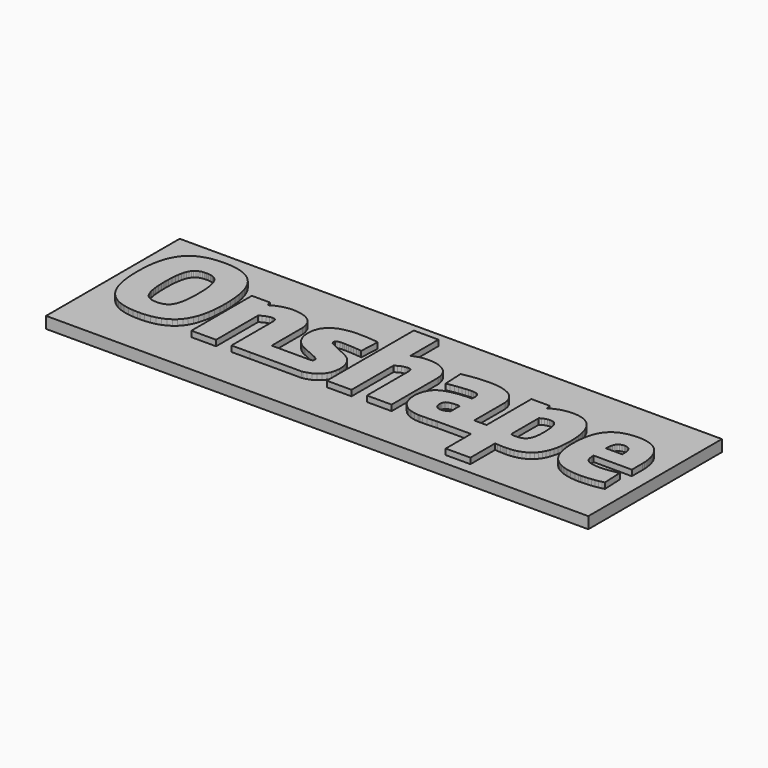
from build123d import *

# Parameters (mm, degrees)
F4_DEPTH = 21.0730088496
F3_W     = 659.7553988
F3_H     = 203.2
F5_DEPTH = 14.0486725664
F6_SCALE = 0.226


# Not quite as in the source:
# - a length typed as a fraction of an inch, garbled in the dataset ("3 / 203.2 mm" for 3/8 in), is restored


with BuildPart() as f4:
    # F3 (on Top) → F4 (new body)
    with BuildSketch(Plane.XY):
        Polygon((-255.4416786, 81.57591), (-257.1904686, 81.57591), (-258.9486566, 81.57591), (-264.2209346, 81.33461), (-270.6951406, 80.60309), (-276.6260406, 79.37881), (-282.0281126, 77.65669), (-286.9158346, 75.43165), (-291.3049546, 72.69861), (-295.2061406, 69.44995), (-298.637579, 65.68567), (-301.6113856, 61.39561), (-304.1428258, 56.57977), (-306.2443456, 51.22799), (-307.9324296, 45.34281), (-309.2209208, 38.91153), (-310.1235352, 31.93415), (-310.654065, 24.40305), (-310.8276994, 18.33753), (-310.8276994, 16.31315), (-310.8276994, 14.29131), (-310.654065, 8.22833), (-310.1235352, 0.70231), (-309.2209208, -6.26491), (-307.9324296, -12.68603), (-306.2443456, -18.55851), (-304.1428258, -23.88997), (-301.6113856, -28.69057), (-298.637579, -32.96285), (-295.2061406, -36.70935), (-291.3049546, -39.94023), (-286.9158346, -42.65803), (-282.0281126, -44.86783), (-276.6260406, -46.57979), (-270.6951406, -47.79645), (-264.2209346, -48.52035), (-258.9486566, -48.75911), (-257.1904686, -48.75911), (-255.4416786, -48.75911), (-250.1953086, -48.52035), (-243.7569166, -47.79645), (-237.8608146, -46.57979), (-232.4917626, -44.86783), (-227.6355366, -42.65803), (-223.2781666, -39.94023), (-219.4059366, -36.70935), (-216.0023366, -32.96285), (-213.0531426, -28.69057), (-210.5451466, -23.88997), (-208.4631086, -18.55851), (-206.7912806, -12.68603), (-205.5167086, -6.26491), (-204.6251686, 0.70231), (-204.0998966, 8.22833), (-203.9276846, 14.29131), (-203.9276846, 16.31315), (-203.9276846, 18.33753), (-204.0998966, 24.40305), (-204.6251686, 31.93415), (-205.5167086, 38.91153), (-206.7912806, 45.34281), (-208.4631086, 51.22799), (-210.5451466, 56.57977), (-213.0531426, 61.39561), (-216.0023366, 65.68567), (-219.4059366, 69.44995), (-223.2781666, 72.69861), (-227.6355366, 75.43165), (-232.4917626, 77.65669), (-237.8608146, 79.37881), (-243.7569166, 80.60309), (-250.1953086, 81.33461), align=None)
        Polygon((-256.5633426, -21.56841), (-257.1904686, -21.56841), (-257.8269926, -21.56841), (-259.7342786, -21.48205), (-262.0906366, -21.20773), (-264.2651306, -20.72513), (-266.2592846, -20.00123), (-268.0769086, -19.01317), (-269.7207966, -17.74063), (-271.1924726, -16.15313), (-272.4975246, -14.23035), (-273.6387466, -11.94435), (-274.6156306, -9.26973), (-275.4352886, -6.18363), (-276.0997526, -2.65811), (-276.6095306, 1.32715), (-276.9707186, 5.80517), (-277.1856026, 10.78865), (-277.2557066, 14.93393), (-277.2557066, 16.31315), (-277.2557066, 17.69745), (-277.1856026, 21.84019), (-276.9707186, 26.83383), (-276.6095306, 31.31947), (-276.0997526, 35.31743), (-275.4352886, 38.85565), (-274.6156306, 41.95953), (-273.6387466, 44.64939), (-272.4975246, 46.95571), (-271.1924726, 48.89627), (-269.7207966, 50.49647), (-268.0769086, 51.78933), (-266.2592846, 52.79009), (-264.2651306, 53.52415), (-262.0906366, 54.01945), (-259.7342786, 54.29631), (-257.8269926, 54.38521), (-257.1904686, 54.38521), (-256.5633426, 54.38521), (-254.6779006, 54.30139), (-252.3436406, 54.02453), (-250.1856566, 53.53939), (-248.1998846, 52.81549), (-246.3865786, 51.82489), (-244.7424366, 50.54727), (-243.2651726, 48.95469), (-241.9519926, 47.02683), (-240.8023886, 44.73067), (-239.8133126, 42.04081), (-238.9822246, 38.93947), (-238.3070926, 35.39617), (-237.7861386, 31.38805), (-237.4168226, 26.88971), (-237.1963506, 21.87321), (-237.1234526, 17.70253), (-237.1234526, 16.31315), (-237.1234526, 14.92631), (-237.1963506, 10.75817), (-237.4168226, 5.74675), (-237.7861386, 1.25603), (-238.3070926, -2.73685), (-238.9822246, -6.26491), (-239.8133126, -9.35101), (-240.8023886, -12.02055), (-241.9519926, -14.30147), (-243.2651726, -16.21663), (-244.7424366, -17.78889), (-246.3865786, -19.05381), (-248.1998846, -20.02663), (-250.1856566, -20.73783), (-252.3436406, -21.21789), (-254.6779006, -21.48205), align=None, mode=Mode.SUBTRACT)
    extrude(amount=F4_DEPTH)



with BuildPart() as f4b:
    # F3 (on Top) → F4, piece 2 (new body)
    with BuildSketch(Plane.XY):
        Polygon((-50.1012206, 5.24383), (-50.9191006, 5.62483), (-70.0513966, 14.62659), (-70.5279006, 14.84503), (-71.9403946, 15.54353), (-73.3544126, 16.47825), (-74.2421426, 17.66189), (-74.5479586, 18.90141), (-74.5479586, 19.31543), (-74.5479586, 19.75993), (-74.1148886, 21.09089), (-72.6284806, 22.24659), (-69.8040006, 22.87397), (-66.4715206, 23.06447), (-65.3615406, 23.06447), (-65.0237206, 23.06447), (-64.0026406, 23.04669), (-61.8690406, 22.98827), (-59.1360006, 22.87905), (-55.9838606, 22.71649), (-52.5853406, 22.49043), (-49.1157006, 22.19833), (-45.7527406, 21.82749), (-43.4362606, 21.50999), (-42.6691806, 21.38045), (-41.5439606, 45.19549), (-42.3059606, 45.32503), (-44.5995806, 45.64761), (-47.9142806, 46.01337), (-51.3610606, 46.30547), (-54.8129206, 46.53153), (-58.1403206, 46.69409), (-61.2188006, 46.80331), (-63.9188206, 46.86427), (-65.5622006, 46.88205), (-66.1108406, 46.88205), (-68.1606206, 46.88205), (-74.3025946, 46.52137), (-81.7783226, 45.38853), (-88.4247406, 43.42003), (-94.1227226, 40.55745), (-98.7587306, 36.71697), (-102.2133846, 31.85033), (-104.3726386, 25.88387), (-105.1168586, 20.53717), (-105.1168586, 18.75155), (-105.1168586, 17.49933), (-104.7681166, 13.73759), (-103.7663406, 9.23671), (-102.1803646, 5.23367), (-100.0772446, 1.71069), (-97.5253066, -1.34747), (-94.5941466, -3.95351), (-91.3503126, -6.12267), (-88.7567186, -7.49173), (-87.8623846, -7.87781), (-70.6122286, -15.56639), (-70.0513966, -15.81531), (-68.4273206, -16.69669), (-66.9084006, -17.86255), (-66.0244806, -19.10207), (-65.7374606, -20.10791), (-65.7374606, -20.44319), (-65.7374606, -20.68957), (-65.8314406, -21.42617), (-66.1337006, -22.15769), (-66.6823406, -22.66823), (-67.5129206, -23.00097), (-68.6610006, -23.19401), (-70.1588386, -23.28545), (-72.0452966, -23.31085), (-73.7773226, -23.31085), (-74.3533946, -23.31085), (-75.5360186, -23.31085), (-79.0790646, -23.31085), (-85.2952066, -23.31085), (-92.4722306, -23.31339), (-98.1758006, -23.31847), (-100.0759746, -23.32101), (-100.0759746, -23.31085), (-115.8120366, -23.31085), (-115.8120366, 22.12721), (-115.8120366, 23.76805), (-116.5024086, 28.68549), (-118.4493186, 34.06521), (-121.4686166, 38.36797), (-125.3769146, 41.68267), (-129.9875226, 44.09567), (-135.1165446, 45.70603), (-140.5808466, 46.60265), (-144.7906426, 46.88205), (-146.1934846, 46.88205), (-147.9712306, 46.88205), (-153.3026906, 46.28769), (-159.8840846, 44.65447), (-165.7631686, 42.21353), (-169.5787566, 40.04437), (-170.7598566, 39.19347), (-170.9485786, 39.19347), (-172.6338686, 45.00499), (-194.5776906, 45.00499), (-194.5776906, -46.88205), (-164.5711466, -46.88205), (-164.5711466, 16.87703), (-163.7926366, 17.44599), (-161.3021666, 18.93443), (-157.8200806, 20.53717), (-154.3392646, 21.57349), (-151.8863866, 21.93925), (-151.0674906, 21.93925), (-150.7421166, 21.93925), (-149.7654866, 21.87067), (-148.6656666, 21.64969), (-147.7588866, 21.26869), (-147.0367646, 20.72259), (-146.4899026, 19.99869), (-146.1106806, 19.09445), (-145.8902086, 17.99209), (-145.8170566, 17.01927), (-145.8170566, 16.69161), (-145.8170566, -46.88205), (-123.4378786, -46.88205), (-60.4542606, -46.92523), (-59.1131406, -46.68901), (-55.1405806, -45.67047), (-50.3272806, -43.85183), (-46.0753206, -41.43629), (-42.4558206, -38.38829), (-39.5272006, -34.66973), (-37.3529606, -30.24759), (-36.0042206, -25.07869), (-35.5394006, -20.61591), (-35.5394006, -19.13001), (-35.5394006, -17.97685), (-35.8391206, -14.51991), (-36.7027206, -10.38479), (-38.0819406, -6.69925), (-39.9234406, -3.44551), (-42.1815006, -0.60579), (-44.7977006, 1.83769), (-47.7288606, 3.91033), align=None)
    extrude(amount=F4_DEPTH)


with BuildPart() as f4c:
    # F3 (on Top) → F4, piece 3 (new body)
    with BuildSketch(Plane.XY):
        Polygon((19.9824594, 46.88459), (18.5778394, 46.88459), (17.3408594, 46.88459), (13.6248394, 46.57725), (8.7785194, 45.71365), (4.2827194, 44.35221), (1.3185394, 43.09237), (0.3863594, 42.57167), (0.1983994, 42.57167), (0.1983994, 85.33003), (-29.8091606, 85.33003), (-29.8091606, -46.88205), (0.1983994, -46.88205), (0.1983994, 16.87703), (0.9781794, 17.44599), (3.4673794, 18.93443), (6.9497194, 20.53717), (10.4295194, 21.57349), (12.8806194, 21.93925), (13.7010394, 21.93925), (14.0261594, 21.93925), (15.0015194, 21.87067), (16.1013394, 21.64969), (17.0106594, 21.26869), (17.7320194, 20.72259), (18.2781194, 19.99869), (18.6591194, 19.09445), (18.8800994, 17.99717), (18.9512194, 17.01927), (18.9512194, 16.69161), (18.9512194, -46.88205), (48.9613194, -46.88205), (48.9613194, 22.12721), (48.9613194, 23.76805), (48.2678994, 28.68549), (46.3222594, 34.06521), (43.3021994, 38.36797), (39.3931394, 41.68267), (34.7830394, 44.09567), (29.6522394, 45.70603), (24.1912394, 46.60519), align=None)
    extrude(amount=F4_DEPTH)


with BuildPart() as f4d:
    # F3 (on Top) → F4, piece 4 (new body)
    with BuildSketch(Plane.XY):
        Polygon((196.4946794, 46.88459), (195.2983394, 46.88459), (193.6498794, 46.88459), (188.6994194, 46.50105), (181.8668194, 45.22089), (175.2831394, 42.84853), (170.7466994, 40.27805), (169.4208194, 39.19347), (169.2328594, 39.19347), (167.5437594, 45.00753), (145.6006994, 45.00753), (145.6006994, -23.32101), (130.5969194, -23.32101), (130.5969194, 21.75383), (130.5969194, 23.36927), (129.8171394, 28.21559), (127.5870194, 33.59277), (124.0818194, 37.94633), (119.4640994, 41.34993), (113.9040394, 43.87977), (107.5743594, 45.59427), (100.6426994, 46.57471), (95.1181994, 46.88459), (93.2766994, 46.88459), (91.5469594, 46.88459), (86.3628194, 46.66615), (78.1763994, 45.99305), (69.4362594, 44.82465), (62.9617994, 43.63847), (60.8307394, 43.13047), (61.9559594, 18.94205), (63.1268994, 19.18843), (66.6651194, 19.84883), (71.3133194, 20.60321), (75.7862594, 21.22043), (79.9823394, 21.70811), (83.8050394, 22.06625), (87.1451394, 22.31517), (89.8959594, 22.45995), (91.4478994, 22.50059), (91.9635194, 22.50059), (92.9312594, 22.50059), (95.8243194, 22.18309), (98.6462594, 21.07565), (100.3785394, 18.94459), (100.9678194, 16.40967), (100.9678194, 15.56639), (100.9678194, 10.49909), (99.6216194, 10.49909), (95.5982594, 10.40511), (90.0102594, 10.09015), (84.3765394, 9.50595), (78.8571194, 8.60425), (73.6323394, 7.34187), (68.8672994, 5.67817), (64.7321794, 3.55727), (62.1413794, 1.68275), (61.3946194, 0.93599), (60.4116394, -0.04445), (57.9554594, -3.49123), (55.6948594, -8.46201), (54.4553394, -13.75029), (54.0794194, -17.78635), (54.0794194, -19.13001), (54.0794194, -20.80133), (54.6585394, -25.83053), (56.3222394, -31.59125), (58.9663794, -36.43503), (62.4715794, -40.37711), (66.7362394, -43.44035), (71.6435194, -45.64253), (77.0867394, -46.99635), (81.4910994, -47.49419), (82.9617594, -47.52467), (83.9980794, -47.54245), (87.1095794, -47.53229), (92.3343594, -47.42307), (98.3312994, -47.20463), (103.1750794, -46.97095), (104.7879794, -46.87951), (145.6006994, -46.88967), (145.6006994, -85.33003), (175.6082594, -85.33003), (175.6082594, -47.63389), (176.3829594, -47.75073), (178.7400794, -47.99203), (182.2655994, -48.22063), (185.7885794, -48.34763), (188.1380794, -48.38573), (188.9254794, -48.38573), (190.1573794, -48.38573), (193.8505394, -48.20031), (198.4403194, -47.63897), (202.6897394, -46.69917), (206.6089594, -45.38853), (210.1979794, -43.69689), (213.4542594, -41.62933), (216.3930394, -39.18585), (219.0016194, -36.35883), (221.2952394, -33.15335), (223.2738994, -29.56941), (224.9401394, -25.59939), (226.2939594, -21.25091), (227.3455194, -16.51381), (228.0897394, -11.39317), (228.5342394, -5.89153), (228.6866394, -1.47447), (228.6866394, -0.00381), (228.6866394, 1.17475), (228.6053594, 4.69519), (228.3513594, 9.28243), (227.8992394, 13.72743), (227.2413794, 18.00733), (226.3447594, 22.09165), (225.1915994, 25.95753), (223.7691994, 29.58211), (222.0470794, 32.93745), (220.0150794, 35.99053), (217.6477994, 38.72611), (214.9249194, 41.11117), (211.8311994, 43.12031), (208.3386994, 44.72559), (204.4321794, 45.90669), (200.0938594, 46.63567), align=None)
        Polygon((101.3361194, -8.62711), (101.3361194, -22.50567), (100.8890794, -22.91461), (99.3193594, -23.90267), (96.8606394, -24.96439), (94.3003194, -25.64257), (92.5451794, -25.88133), (91.9635194, -25.88133), (91.0465794, -25.88133), (88.2982994, -25.31745), (85.7278194, -23.63089), (84.2063594, -20.81657), (83.7085194, -17.86255), (83.7085194, -16.87957), (83.7085194, -16.62557), (83.7643994, -15.87119), (84.0158594, -14.44117), (84.5797394, -12.86891), (85.2833194, -11.74369), (85.5855794, -11.43889), (86.1011994, -10.92581), (88.1535194, -9.89203), (91.7730194, -9.04875), (96.2408794, -8.69823), (100.0635794, -8.62711), align=None, mode=Mode.SUBTRACT)
        Polygon((185.2780394, -24.04745), (184.4245994, -24.12619), (183.8835794, -24.17191), (182.2579794, -24.21255), (179.8805394, -24.12873), (177.5665994, -23.86203), (176.0806994, -23.55723), (175.6082594, -23.39975), (175.6082594, 18.56867), (176.1060994, 18.95221), (177.7342394, 19.94281), (180.3885394, 21.14677), (183.4670194, 21.99767), (186.0146394, 22.31771), (186.8604594, 22.31771), (187.4878394, 22.31771), (189.3648994, 22.10181), (191.5391394, 21.36775), (193.3780994, 19.98599), (194.8766994, 17.81683), (196.0476394, 14.73581), (196.8807594, 10.60831), (197.3811394, 5.30225), (197.5462394, 0.33909), (197.5462394, -1.31445), (197.5462394, -2.68097), (197.3887594, -6.78053), (196.8832994, -11.40079), (195.9942994, -15.22603), (194.6811194, -18.30197), (192.9107394, -20.67941), (190.6348994, -22.40661), (187.8180394, -23.53945), align=None, mode=Mode.SUBTRACT)
    extrude(amount=F4_DEPTH)


with BuildPart() as f4e:
    # F3 (on Top) → F4, piece 5 (new body)
    with BuildSketch(Plane.XY):
        Polygon((276.0119194, 46.88459), (274.8181194, 46.88459), (273.3982594, 46.88459), (269.1285194, 46.67377), (263.9316794, 46.04893), (259.2098194, 45.01515), (254.9426194, 43.58005), (251.1199194, 41.74871), (247.7188594, 39.52621), (244.7241994, 36.92271), (242.1156194, 33.94583), (239.8829594, 30.59811), (238.0033594, 26.88717), (236.4590394, 22.81809), (235.2347594, 18.40103), (234.3127394, 13.64361), (233.6751994, 8.54837), (233.3043594, 3.12293), (233.1849794, -1.19253), (233.1849794, -2.62763), (233.1849794, -3.94081), (233.3221394, -7.87273), (233.7463194, -12.84859), (234.4727594, -17.53997), (235.5166994, -21.93925), (236.9035394, -26.03881), (238.6459794, -29.83103), (240.7592594, -33.30575), (243.2662394, -36.45281), (246.1796194, -39.26459), (249.5222594, -41.72839), (253.3068594, -43.83913), (257.5537394, -45.58411), (262.2806794, -46.96079), (267.5029194, -47.95647), (273.2382394, -48.55591), (277.9423194, -48.75911), (279.5069594, -48.75911), (280.1927594, -48.75911), (282.2374594, -48.70831), (285.5343794, -48.54575), (289.2122994, -48.27651), (293.1035794, -47.89297), (297.0304194, -47.39513), (300.8200994, -46.78045), (304.2871994, -46.05147), (306.5300194, -45.44695), (307.2640794, -45.20057), (306.1363194, -21.19503), (304.9780794, -21.52269), (301.4474794, -22.32279), (295.7527994, -23.34895), (289.8117394, -24.09317), (285.7401194, -24.38273), (284.3837594, -24.38273), (282.8495994, -24.38273), (278.2445794, -24.12873), (273.4973194, -23.37435), (269.9590994, -22.12467), (267.4571994, -20.39747), (265.8188994, -18.18767), (264.8663994, -15.51813), (264.4218994, -12.39139), (264.3177594, -9.70661), (264.3177594, -8.81507), (310.8276994, -8.81507), (310.8276994, 6.56209), (310.8276994, 7.61619), (310.7133994, 10.78611), (310.3654194, 14.86281), (309.7685194, 18.77949), (308.9176194, 22.51583), (307.8000194, 26.05405), (306.4080994, 29.37637), (304.7240794, 32.46755), (302.7377994, 35.30219), (300.4441794, 37.87521), (297.8305194, 40.15867), (294.8891994, 42.13987), (291.5998994, 43.80103), (287.9600794, 45.12437), (283.9595794, 46.09211), (279.5806194, 46.68393), align=None)
        Polygon((284.0129194, 11.81481), (284.0129194, 10.12571), (264.1297994, 10.12571), (264.1628194, 10.91311), (264.3279194, 13.26515), (264.6936794, 16.16837), (265.3108994, 18.78203), (266.2608594, 21.05025), (267.6248394, 22.91461), (269.4815794, 24.31415), (271.9148994, 25.19553), (274.2339194, 25.50287), (275.0086194, 25.50287), (275.6563194, 25.50287), (277.6019594, 25.19299), (279.6568194, 24.31415), (281.2366994, 22.95271), (282.3923994, 21.19249), (283.1899594, 19.11477), (283.6852594, 16.80337), (283.9417994, 14.34211), (284.0129194, 12.44727), align=None, mode=Mode.SUBTRACT)
    extrude(amount=F4_DEPTH)


with BuildPart() as f4_1:
    add(f4.part)

    add(f4b.part)  # F5 merges F4b

    add(f4c.part)  # F5 merges F4c

    add(f4d.part)  # F5 merges F4d

    add(f4e.part)  # F5 merges F4e
    # F3 (on Top) → F5 (join)
    with BuildSketch(Plane.XY):
        with Locations((0, 2.78003)):
            Rectangle(F3_W, F3_H)
        Polygon((-70.0513966, 14.62659), (-50.9191006, 5.62483), (-50.1012206, 5.24383), (-47.7288606, 3.91033), (-44.7977006, 1.83769), (-42.1815006, -0.60579), (-39.9234406, -3.44551), (-38.0819406, -6.69925), (-36.7027206, -10.38479), (-35.8391206, -14.51991), (-35.5394006, -17.97685), (-35.5394006, -19.13001), (-35.5394006, -20.61591), (-36.0042206, -25.07869), (-37.3529606, -30.24759), (-39.5272006, -34.66973), (-42.4558206, -38.38829), (-46.0753206, -41.43629), (-50.3272806, -43.85183), (-55.1405806, -45.67047), (-59.1131406, -46.68901), (-60.4542606, -46.92523), (-123.4378786, -46.88205), (-145.8170566, -46.88205), (-145.8170566, 16.69161), (-145.8170566, 17.01927), (-145.8902086, 17.99209), (-146.1106806, 19.09445), (-146.4899026, 19.99869), (-147.0367646, 20.72259), (-147.7588866, 21.26869), (-148.6656666, 21.64969), (-149.7654866, 21.87067), (-150.7421166, 21.93925), (-151.0674906, 21.93925), (-151.8863866, 21.93925), (-154.3392646, 21.57349), (-157.8200806, 20.53717), (-161.3021666, 18.93443), (-163.7926366, 17.44599), (-164.5711466, 16.87703), (-164.5711466, -46.88205), (-194.5776906, -46.88205), (-194.5776906, 45.00499), (-172.6338686, 45.00499), (-170.9485786, 39.19347), (-170.7598566, 39.19347), (-169.5787566, 40.04437), (-165.7631686, 42.21353), (-159.8840846, 44.65447), (-153.3026906, 46.28769), (-147.9712306, 46.88205), (-146.1934846, 46.88205), (-144.7906426, 46.88205), (-140.5808466, 46.60265), (-135.1165446, 45.70603), (-129.9875226, 44.09567), (-125.3769146, 41.68267), (-121.4686166, 38.36797), (-118.4493186, 34.06521), (-116.5024086, 28.68549), (-115.8120366, 23.76805), (-115.8120366, 22.12721), (-115.8120366, -23.31085), (-100.0759746, -23.31085), (-100.0759746, -23.32101), (-98.1758006, -23.31847), (-92.4722306, -23.31339), (-85.2952066, -23.31085), (-79.0790646, -23.31085), (-75.5360186, -23.31085), (-74.3533946, -23.31085), (-73.7773226, -23.31085), (-72.0452966, -23.31085), (-70.1588386, -23.28545), (-68.6610006, -23.19401), (-67.5129206, -23.00097), (-66.6823406, -22.66823), (-66.1337006, -22.15769), (-65.8314406, -21.42617), (-65.7374606, -20.68957), (-65.7374606, -20.44319), (-65.7374606, -20.10791), (-66.0244806, -19.10207), (-66.9084006, -17.86255), (-68.4273206, -16.69669), (-70.0513966, -15.81531), (-70.6122286, -15.56639), (-87.8623846, -7.87781), (-88.7567186, -7.49173), (-91.3503126, -6.12267), (-94.5941466, -3.95351), (-97.5253066, -1.34747), (-100.0772446, 1.71069), (-102.1803646, 5.23367), (-103.7663406, 9.23671), (-104.7681166, 13.73759), (-105.1168586, 17.49933), (-105.1168586, 18.75155), (-105.1168586, 20.53717), (-104.3726386, 25.88387), (-102.2133846, 31.85033), (-98.7587306, 36.71697), (-94.1227226, 40.55745), (-88.4247406, 43.42003), (-81.7783226, 45.38853), (-74.3025946, 46.52137), (-68.1606206, 46.88205), (-66.1108406, 46.88205), (-65.5622006, 46.88205), (-63.9188206, 46.86427), (-61.2188006, 46.80331), (-58.1403206, 46.69409), (-54.8129206, 46.53153), (-51.3610606, 46.30547), (-47.9142806, 46.01337), (-44.5995806, 45.64761), (-42.3059606, 45.32503), (-41.5439606, 45.19549), (-42.6691806, 21.38045), (-43.4362606, 21.50999), (-45.7527406, 21.82749), (-49.1157006, 22.19833), (-52.5853406, 22.49043), (-55.9838606, 22.71649), (-59.1360006, 22.87905), (-61.8690406, 22.98827), (-64.0026406, 23.04669), (-65.0237206, 23.06447), (-65.3615406, 23.06447), (-66.4715206, 23.06447), (-69.8040006, 22.87397), (-72.6284806, 22.24659), (-74.1148886, 21.09089), (-74.5479586, 19.75993), (-74.5479586, 19.31543), (-74.5479586, 18.90141), (-74.2421426, 17.66189), (-73.3544126, 16.47825), (-71.9403946, 15.54353), (-70.5279006, 14.84503), align=None, mode=Mode.SUBTRACT)
        Polygon((193.6498794, 46.88459), (195.2983394, 46.88459), (196.4946794, 46.88459), (200.0938594, 46.63567), (204.4321794, 45.90669), (208.3386994, 44.72559), (211.8311994, 43.12031), (214.9249194, 41.11117), (217.6477994, 38.72611), (220.0150794, 35.99053), (222.0470794, 32.93745), (223.7691994, 29.58211), (225.1915994, 25.95753), (226.3447594, 22.09165), (227.2413794, 18.00733), (227.8992394, 13.72743), (228.3513594, 9.28243), (228.6053594, 4.69519), (228.6866394, 1.17475), (228.6866394, -0.00381), (228.6866394, -1.47447), (228.5342394, -5.89153), (228.0897394, -11.39317), (227.3455194, -16.51381), (226.2939594, -21.25091), (224.9401394, -25.59939), (223.2738994, -29.56941), (221.2952394, -33.15335), (219.0016194, -36.35883), (216.3930394, -39.18585), (213.4542594, -41.62933), (210.1979794, -43.69689), (206.6089594, -45.38853), (202.6897394, -46.69917), (198.4403194, -47.63897), (193.8505394, -48.20031), (190.1573794, -48.38573), (188.9254794, -48.38573), (188.1380794, -48.38573), (185.7885794, -48.34763), (182.2655994, -48.22063), (178.7400794, -47.99203), (176.3829594, -47.75073), (175.6082594, -47.63389), (175.6082594, -85.33003), (145.6006994, -85.33003), (145.6006994, -46.88967), (104.7879794, -46.87951), (103.1750794, -46.97095), (98.3312994, -47.20463), (92.3343594, -47.42307), (87.1095794, -47.53229), (83.9980794, -47.54245), (82.9617594, -47.52467), (81.4910994, -47.49419), (77.0867394, -46.99635), (71.6435194, -45.64253), (66.7362394, -43.44035), (62.4715794, -40.37711), (58.9663794, -36.43503), (56.3222394, -31.59125), (54.6585394, -25.83053), (54.0794194, -20.80133), (54.0794194, -19.13001), (54.0794194, -17.78635), (54.4553394, -13.75029), (55.6948594, -8.46201), (57.9554594, -3.49123), (60.4116394, -0.04445), (61.3946194, 0.93599), (62.1413794, 1.68275), (64.7321794, 3.55727), (68.8672994, 5.67817), (73.6323394, 7.34187), (78.8571194, 8.60425), (84.3765394, 9.50595), (90.0102594, 10.09015), (95.5982594, 10.40511), (99.6216194, 10.49909), (100.9678194, 10.49909), (100.9678194, 15.56639), (100.9678194, 16.40967), (100.3785394, 18.94459), (98.6462594, 21.07565), (95.8243194, 22.18309), (92.9312594, 22.50059), (91.9635194, 22.50059), (91.4478994, 22.50059), (89.8959594, 22.45995), (87.1451394, 22.31517), (83.8050394, 22.06625), (79.9823394, 21.70811), (75.7862594, 21.22043), (71.3133194, 20.60321), (66.6651194, 19.84883), (63.1268994, 19.18843), (61.9559594, 18.94205), (60.8307394, 43.13047), (62.9617994, 43.63847), (69.4362594, 44.82465), (78.1763994, 45.99305), (86.3628194, 46.66615), (91.5469594, 46.88459), (93.2766994, 46.88459), (95.1181994, 46.88459), (100.6426994, 46.57471), (107.5743594, 45.59427), (113.9040394, 43.87977), (119.4640994, 41.34993), (124.0818194, 37.94633), (127.5870194, 33.59277), (129.8171394, 28.21559), (130.5969194, 23.36927), (130.5969194, 21.75383), (130.5969194, -23.32101), (145.6006994, -23.32101), (145.6006994, 45.00753), (167.5437594, 45.00753), (169.2328594, 39.19347), (169.4208194, 39.19347), (170.7466994, 40.27805), (175.2831394, 42.84853), (181.8668194, 45.22089), (188.6994194, 46.50105), align=None, mode=Mode.SUBTRACT)
        Polygon((273.3982594, 46.88459), (274.8181194, 46.88459), (276.0119194, 46.88459), (279.5806194, 46.68393), (283.9595794, 46.09211), (287.9600794, 45.12437), (291.5998994, 43.80103), (294.8891994, 42.13987), (297.8305194, 40.15867), (300.4441794, 37.87521), (302.7377994, 35.30219), (304.7240794, 32.46755), (306.4080994, 29.37637), (307.8000194, 26.05405), (308.9176194, 22.51583), (309.7685194, 18.77949), (310.3654194, 14.86281), (310.7133994, 10.78611), (310.8276994, 7.61619), (310.8276994, 6.56209), (310.8276994, -8.81507), (264.3177594, -8.81507), (264.3177594, -9.70661), (264.4218994, -12.39139), (264.8663994, -15.51813), (265.8188994, -18.18767), (267.4571994, -20.39747), (269.9590994, -22.12467), (273.4973194, -23.37435), (278.2445794, -24.12873), (282.8495994, -24.38273), (284.3837594, -24.38273), (285.7401194, -24.38273), (289.8117394, -24.09317), (295.7527994, -23.34895), (301.4474794, -22.32279), (304.9780794, -21.52269), (306.1363194, -21.19503), (307.2640794, -45.20057), (306.5300194, -45.44695), (304.2871994, -46.05147), (300.8200994, -46.78045), (297.0304194, -47.39513), (293.1035794, -47.89297), (289.2122994, -48.27651), (285.5343794, -48.54575), (282.2374594, -48.70831), (280.1927594, -48.75911), (279.5069594, -48.75911), (277.9423194, -48.75911), (273.2382394, -48.55591), (267.5029194, -47.95647), (262.2806794, -46.96079), (257.5537394, -45.58411), (253.3068594, -43.83913), (249.5222594, -41.72839), (246.1796194, -39.26459), (243.2662394, -36.45281), (240.7592594, -33.30575), (238.6459794, -29.83103), (236.9035394, -26.03881), (235.5166994, -21.93925), (234.4727594, -17.53997), (233.7463194, -12.84859), (233.3221394, -7.87273), (233.1849794, -3.94081), (233.1849794, -2.62763), (233.1849794, -1.19253), (233.3043594, 3.12293), (233.6751994, 8.54837), (234.3127394, 13.64361), (235.2347594, 18.40103), (236.4590394, 22.81809), (238.0033594, 26.88717), (239.8829594, 30.59811), (242.1156194, 33.94583), (244.7241994, 36.92271), (247.7188594, 39.52621), (251.1199194, 41.74871), (254.9426194, 43.58005), (259.2098194, 45.01515), (263.9316794, 46.04893), (269.1285194, 46.67377), align=None, mode=Mode.SUBTRACT)
        Polygon((-258.9486566, 81.57591), (-257.1904686, 81.57591), (-255.4416786, 81.57591), (-250.1953086, 81.33461), (-243.7569166, 80.60309), (-237.8608146, 79.37881), (-232.4917626, 77.65669), (-227.6355366, 75.43165), (-223.2781666, 72.69861), (-219.4059366, 69.44995), (-216.0023366, 65.68567), (-213.0531426, 61.39561), (-210.5451466, 56.57977), (-208.4631086, 51.22799), (-206.7912806, 45.34281), (-205.5167086, 38.91153), (-204.6251686, 31.93415), (-204.0998966, 24.40305), (-203.9276846, 18.33753), (-203.9276846, 16.31315), (-203.9276846, 14.29131), (-204.0998966, 8.22833), (-204.6251686, 0.70231), (-205.5167086, -6.26491), (-206.7912806, -12.68603), (-208.4631086, -18.55851), (-210.5451466, -23.88997), (-213.0531426, -28.69057), (-216.0023366, -32.96285), (-219.4059366, -36.70935), (-223.2781666, -39.94023), (-227.6355366, -42.65803), (-232.4917626, -44.86783), (-237.8608146, -46.57979), (-243.7569166, -47.79645), (-250.1953086, -48.52035), (-255.4416786, -48.75911), (-257.1904686, -48.75911), (-258.9486566, -48.75911), (-264.2209346, -48.52035), (-270.6951406, -47.79645), (-276.6260406, -46.57979), (-282.0281126, -44.86783), (-286.9158346, -42.65803), (-291.3049546, -39.94023), (-295.2061406, -36.70935), (-298.637579, -32.96285), (-301.6113856, -28.69057), (-304.1428258, -23.88997), (-306.2443456, -18.55851), (-307.9324296, -12.68603), (-309.2209208, -6.26491), (-310.1235352, 0.70231), (-310.654065, 8.22833), (-310.8276994, 14.29131), (-310.8276994, 16.31315), (-310.8276994, 18.33753), (-310.654065, 24.40305), (-310.1235352, 31.93415), (-309.2209208, 38.91153), (-307.9324296, 45.34281), (-306.2443456, 51.22799), (-304.1428258, 56.57977), (-301.6113856, 61.39561), (-298.637579, 65.68567), (-295.2061406, 69.44995), (-291.3049546, 72.69861), (-286.9158346, 75.43165), (-282.0281126, 77.65669), (-276.6260406, 79.37881), (-270.6951406, 80.60309), (-264.2209346, 81.33461), align=None, mode=Mode.SUBTRACT)
        Polygon((17.3408594, 46.88459), (18.5778394, 46.88459), (19.9824594, 46.88459), (24.1912394, 46.60519), (29.6522394, 45.70603), (34.7830394, 44.09567), (39.3931394, 41.68267), (43.3021994, 38.36797), (46.3222594, 34.06521), (48.2678994, 28.68549), (48.9613194, 23.76805), (48.9613194, 22.12721), (48.9613194, -46.88205), (18.9512194, -46.88205), (18.9512194, 16.69161), (18.9512194, 17.01927), (18.8800994, 17.99717), (18.6591194, 19.09445), (18.2781194, 19.99869), (17.7320194, 20.72259), (17.0106594, 21.26869), (16.1013394, 21.64969), (15.0015194, 21.87067), (14.0261594, 21.93925), (13.7010394, 21.93925), (12.8806194, 21.93925), (10.4295194, 21.57349), (6.9497194, 20.53717), (3.4673794, 18.93443), (0.9781794, 17.44599), (0.1983994, 16.87703), (0.1983994, -46.88205), (-29.8091606, -46.88205), (-29.8091606, 85.33003), (0.1983994, 85.33003), (0.1983994, 42.57167), (0.3863594, 42.57167), (1.3185394, 43.09237), (4.2827194, 44.35221), (8.7785194, 45.71365), (13.6248394, 46.57725), align=None, mode=Mode.SUBTRACT)
        Polygon((-257.8269926, -21.56841), (-257.1904686, -21.56841), (-256.5633426, -21.56841), (-254.6779006, -21.48205), (-252.3436406, -21.21789), (-250.1856566, -20.73783), (-248.1998846, -20.02663), (-246.3865786, -19.05381), (-244.7424366, -17.78889), (-243.2651726, -16.21663), (-241.9519926, -14.30147), (-240.8023886, -12.02055), (-239.8133126, -9.35101), (-238.9822246, -6.26491), (-238.3070926, -2.73685), (-237.7861386, 1.25603), (-237.4168226, 5.74675), (-237.1963506, 10.75817), (-237.1234526, 14.92631), (-237.1234526, 16.31315), (-237.1234526, 17.70253), (-237.1963506, 21.87321), (-237.4168226, 26.88971), (-237.7861386, 31.38805), (-238.3070926, 35.39617), (-238.9822246, 38.93947), (-239.8133126, 42.04081), (-240.8023886, 44.73067), (-241.9519926, 47.02683), (-243.2651726, 48.95469), (-244.7424366, 50.54727), (-246.3865786, 51.82489), (-248.1998846, 52.81549), (-250.1856566, 53.53939), (-252.3436406, 54.02453), (-254.6779006, 54.30139), (-256.5633426, 54.38521), (-257.1904686, 54.38521), (-257.8269926, 54.38521), (-259.7342786, 54.29631), (-262.0906366, 54.01945), (-264.2651306, 53.52415), (-266.2592846, 52.79009), (-268.0769086, 51.78933), (-269.7207966, 50.49647), (-271.1924726, 48.89627), (-272.4975246, 46.95571), (-273.6387466, 44.64939), (-274.6156306, 41.95953), (-275.4352886, 38.85565), (-276.0997526, 35.31743), (-276.6095306, 31.31947), (-276.9707186, 26.83383), (-277.1856026, 21.84019), (-277.2557066, 17.69745), (-277.2557066, 16.31315), (-277.2557066, 14.93393), (-277.1856026, 10.78865), (-276.9707186, 5.80517), (-276.6095306, 1.32715), (-276.0997526, -2.65811), (-275.4352886, -6.18363), (-274.6156306, -9.26973), (-273.6387466, -11.94435), (-272.4975246, -14.23035), (-271.1924726, -16.15313), (-269.7207966, -17.74063), (-268.0769086, -19.01317), (-266.2592846, -20.00123), (-264.2651306, -20.72513), (-262.0906366, -21.20773), (-259.7342786, -21.48205), align=None)
        Polygon((100.8890794, -22.91461), (101.3361194, -22.50567), (101.3361194, -8.62711), (100.0635794, -8.62711), (96.2408794, -8.69823), (91.7730194, -9.04875), (88.1535194, -9.89203), (86.1011994, -10.92581), (85.5855794, -11.43889), (85.2833194, -11.74369), (84.5797394, -12.86891), (84.0158594, -14.44117), (83.7643994, -15.87119), (83.7085194, -16.62557), (83.7085194, -16.87957), (83.7085194, -17.86255), (84.2063594, -20.81657), (85.7278194, -23.63089), (88.2982994, -25.31745), (91.0465794, -25.88133), (91.9635194, -25.88133), (92.5451794, -25.88133), (94.3003194, -25.64257), (96.8606394, -24.96439), (99.3193594, -23.90267), align=None)
        Polygon((183.8835794, -24.17191), (184.4245994, -24.12619), (185.2780394, -24.04745), (187.8180394, -23.53945), (190.6348994, -22.40661), (192.9107394, -20.67941), (194.6811194, -18.30197), (195.9942994, -15.22603), (196.8832994, -11.40079), (197.3887594, -6.78053), (197.5462394, -2.68097), (197.5462394, -1.31445), (197.5462394, 0.33909), (197.3811394, 5.30225), (196.8807594, 10.60831), (196.0476394, 14.73581), (194.8766994, 17.81683), (193.3780994, 19.98599), (191.5391394, 21.36775), (189.3648994, 22.10181), (187.4878394, 22.31771), (186.8604594, 22.31771), (186.0146394, 22.31771), (183.4670194, 21.99767), (180.3885394, 21.14677), (177.7342394, 19.94281), (176.1060994, 18.95221), (175.6082594, 18.56867), (175.6082594, -23.39975), (176.0806994, -23.55723), (177.5665994, -23.86203), (179.8805394, -24.12873), (182.2579794, -24.21255), align=None)
        Polygon((264.1297994, 10.12571), (284.0129194, 10.12571), (284.0129194, 11.81481), (284.0129194, 12.44727), (283.9417994, 14.34211), (283.6852594, 16.80337), (283.1899594, 19.11477), (282.3923994, 21.19249), (281.2366994, 22.95271), (279.6568194, 24.31415), (277.6019594, 25.19299), (275.6563194, 25.50287), (275.0086194, 25.50287), (274.2339194, 25.50287), (271.9148994, 25.19553), (269.4815794, 24.31415), (267.6248394, 22.91461), (266.2608594, 21.05025), (265.3108994, 18.78203), (264.6936794, 16.16837), (264.3279194, 13.26515), (264.1628194, 10.91311), align=None)
    extrude(amount=F5_DEPTH)


with BuildPart() as f4_2:
    # F6: moved
    add(f4_1.part.scale(F6_SCALE))


solid = f4_2.part
